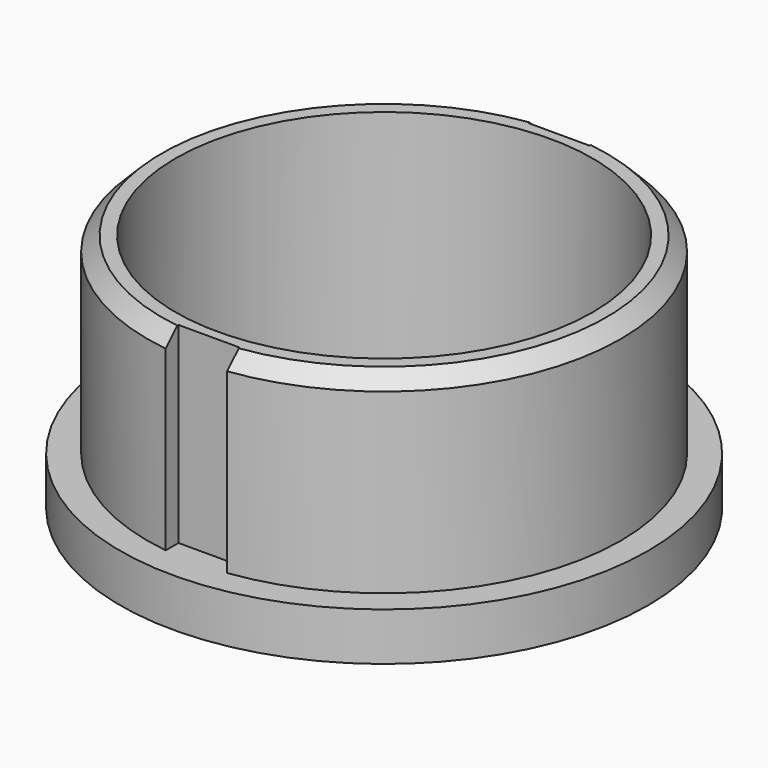
from build123d import *

# Parameters (mm, degrees)
F0_R     = 21.725
F1_DEPTH = 25
F0_R_2   = 27.5
F2_DEPTH = 5
F3_SIZE  = 1.5


# Not quite as in the source:
# - a feature names something its author has since deleted; it is built from what else it names


with BuildPart() as f1:
    # F0 (on Top) → F1 (new body)
    with BuildSketch(Plane.XY):
        with BuildLine():
            Line((-3.2, 22.7763034753), (-3.2, 24.4414095338))
            ThreePointArc((-3.2, 24.4414095338), (-24.65, 0), (-3.2, -24.4414095338))
            Line((-3.2, -24.4414095338), (-3.2, -22.7763034753))
            Line((-3.2, -22.7763034753), (3.2, -22.7763034753))
            Line((3.2, -22.7763034753), (3.2, -24.4414095338))
            ThreePointArc((3.2, -24.4414095338), (24.65, 0), (3.2, 24.4414095338))
            Line((3.2, 24.4414095338), (3.2, 22.7763034753))
            Line((3.2, 22.7763034753), (-3.2, 22.7763034753))
        make_face()
        Circle(F0_R, mode=Mode.SUBTRACT)
    extrude(amount=F1_DEPTH)

    # F0 (on Top) → F2 (join)
    with BuildSketch(Plane.XY):
        Circle(F0_R_2)
        with BuildLine():
            ThreePointArc((-3.2, -24.4414095338), (-24.65, 0), (-3.2, 24.4414095338))
            Line((-3.2, 24.4414095338), (-3.2, 22.7763034753))
            Line((-3.2, 22.7763034753), (3.2, 22.7763034753))
            Line((3.2, 22.7763034753), (3.2, 24.4414095338))
            ThreePointArc((3.2, 24.4414095338), (24.65, 0), (3.2, -24.4414095338))
            Line((3.2, -24.4414095338), (3.2, -22.7763034753))
            Line((3.2, -22.7763034753), (-3.2, -22.7763034753))
            Line((-3.2, -22.7763034753), (-3.2, -24.4414095338))
        make_face(mode=Mode.SUBTRACT)
    extrude(amount=F2_DEPTH)

    # F3
    f3_edges = [f1.edges().sort_by_distance(p)[0] for p in [
        (-24.65, 0, 25),
        (24.65, 0, 25),
        (-21.725, 0, 0),
    ]]
    chamfer(f3_edges, length=F3_SIZE)


solid = f1.part
